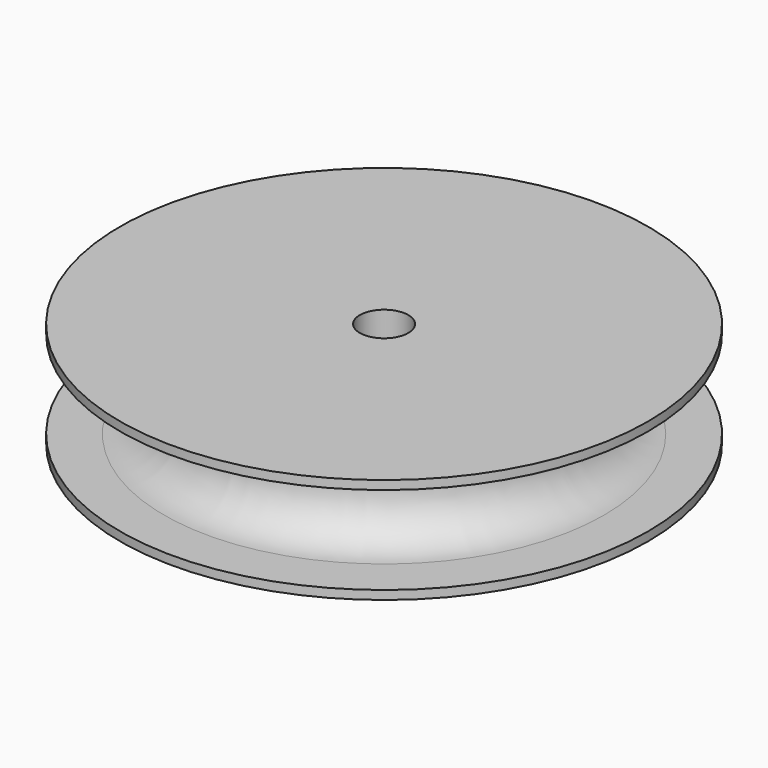
from build123d import *

# Parameters (mm, degrees)
F0_R      = 50.8
F1_DEPTH  = 30.48
F0_R_2    = 76.2
F2_DEPTH  = 2.54
F3_R      = 76.2
F4_DEPTH  = 2.54
F5_R      = 12.69999
F6_R      = 1.27
F7_DEPTH  = 254
F8_DEPTH  = 254
F9_R      = 6.9999987
F10_DEPTH = 27.94


# Not quite as in the source:
# - a fillet or chamfer is up to 0.001 mm smaller than in the source, because OpenCascade refuses the exact size


with BuildPart() as f1:
    # F0 (on Top) → F1 (new body)
    with BuildSketch(Plane.XY):
        Circle(F0_R)
    extrude(amount=F1_DEPTH)

    # F0 (on Top) → F2 (join)
    with BuildSketch(Plane.XY):
        Circle(F0_R_2)
        Circle(F0_R, mode=Mode.SUBTRACT)
    extrude(amount=F2_DEPTH)

    # F3 (on face) → F4 (join)
    with BuildSketch(Plane.XY.offset(30.48)):
        Circle(F3_R)
    extrude(amount=-F4_DEPTH)

    # F5 (radius 12.7 in the source; OpenCascade refuses exactly that, so slightly less here)
    f5_edges = [f1.edges().sort_by_distance(p)[0] for p in [
        (50.8, 0, 15.24),
        (-50.8, 0, 27.94),
        (-50.8, 0, 2.54),
    ]]
    fillet(f5_edges, radius=F5_R)

    # F6 (on Right) → F7 (cut)
    with BuildSketch(Plane.YZ):
        with Locations((0, 15.24)):
            Circle(F6_R)
    extrude(amount=-F7_DEPTH, mode=Mode.SUBTRACT)

    # F6 (on Right) → F8 (cut)
    with BuildSketch(Plane.YZ):
        with Locations((0, 15.24)):
            Circle(F6_R)
    extrude(amount=F8_DEPTH, mode=Mode.SUBTRACT)

    # F9 (on face) → F10 (cut)
    with BuildSketch(Plane.XY.offset(30.48)):
        Circle(F9_R)
    extrude(amount=-F10_DEPTH, mode=Mode.SUBTRACT)


solid = f1.part
